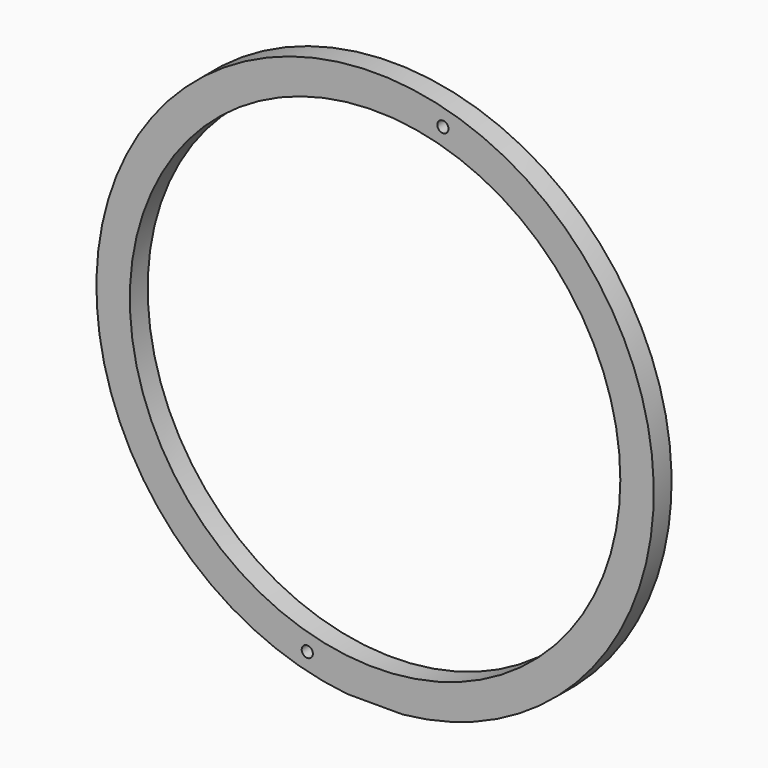
from build123d import *

# Parameters (mm, degrees)
F0_R     = 139.7
F1_DEPTH = 12.7
F6_D     = 6.35
F6_DEPTH = 50.8
F6_TIP   = 1.9077324654


# Not quite as in the source:
# - a pattern or mirror of a feature is missing from the dataset's text; its kind, count and spacing are read off the source's solid


with BuildPart() as f1:
    # F0 (on Front) → F1 (new body)
    with BuildSketch(Plane.XZ):
        with BuildLine():
            ThreePointArc((15.8551438321, -157.95625), (0, 158.75), (-15.8551438321, -157.95625))
            Line((-15.8551438321, -157.95625), (15.8551438321, -157.95625))
        make_face()
        Circle(F0_R, mode=Mode.SUBTRACT)
    extrude(amount=F1_DEPTH)

    # F6
    with Locations(Plane(origin=(0, 0, 0), x_dir=(1, 0, 0), z_dir=(0, 1, 0))):
        with Locations((38.6222720054, -144.140281428)):
            f6 = Hole(F6_D / 2, depth=F6_DEPTH)
            with Locations((0, 0, -(F6_DEPTH + F6_TIP / 2))):  # 118° drill point
                Cone(0, F6_D / 2, F6_TIP, mode=Mode.SUBTRACT)

    # F6_copies: F6 across plane
    add(f6.mirror(Plane(origin=(0, 0, 0), x_dir=(-0.9659258263, 0, 0.2588190451), z_dir=(-0.2588190451, 0, -0.9659258263))), mode=Mode.SUBTRACT)


solid = f1.part
